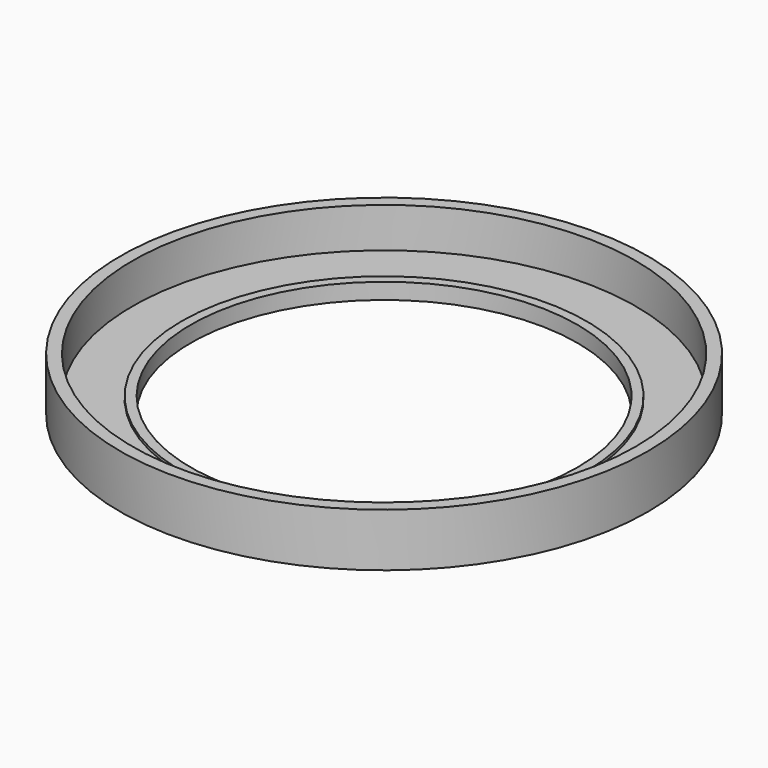
from build123d import *

# Parameters (mm, degrees)
F0_R     = 96.52
F0_R_2   = 92.075
F1_DEPTH = 7.62
F4_R     = 125.73
F4_R_2   = 119.85625
F5_DEPTH = 25.4
F6_R     = 120.65
F6_R_2   = 96.52
F7_DEPTH = 6.35


with BuildPart() as f1:
    # F0 (on Top) → F1 (new body)
    with BuildSketch(Plane.XY):
        Circle(F0_R)
        Circle(F0_R_2, mode=Mode.SUBTRACT)
    extrude(amount=F1_DEPTH)

    # F2 (on Front) → F3 (revolve)
    with BuildSketch(Plane.XZ):
        Polygon((96.52, 2.54), (96.52, 0), (97.79, 0), align=None)
    revolve(axis=Axis((0, 0, 9.845005), (0, 0, 1)))


with BuildPart() as f5:
    # F4 (on Top) → F5 (new body)
    with BuildSketch(Plane.XY):
        Circle(F4_R)
        Circle(F4_R_2, mode=Mode.SUBTRACT)
    extrude(amount=F5_DEPTH)

    # F6 (on Top) → F7 (join)
    with BuildSketch(Plane.XY):
        Circle(F6_R)
        Circle(F6_R_2, mode=Mode.SUBTRACT)
    extrude(amount=F7_DEPTH)


solid = Compound([f1.part, f5.part])
